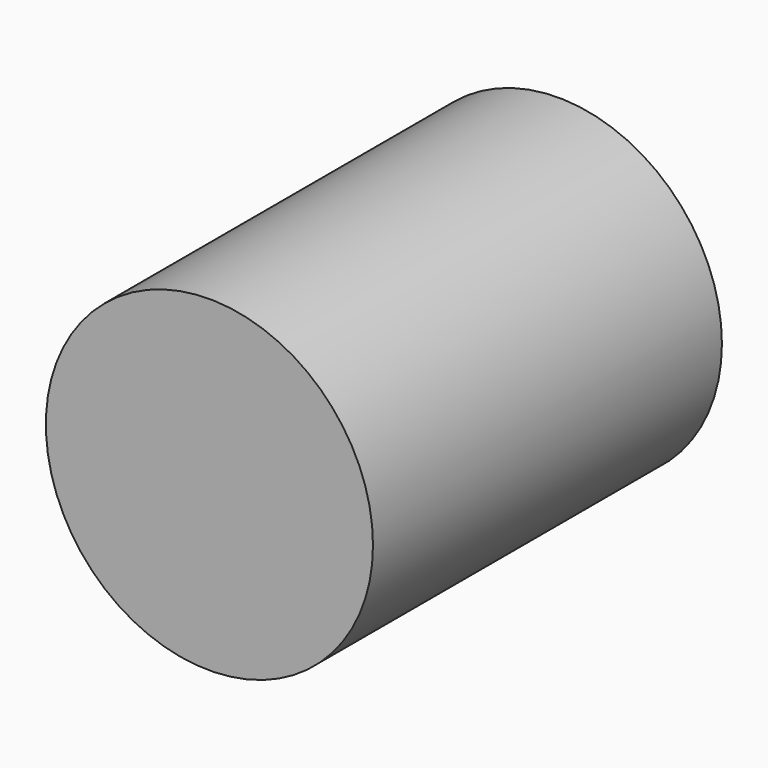
from build123d import *

# Parameters (mm, degrees)
F0_R     = 38.1
F0_R_2   = 19.05
F1_DEPTH = 50.8


# Not quite as in the source:
# - the program builds the solid bodies; features that only make, move or delete a surface that nothing else refers to are left out


with BuildPart() as f1:
    # F0 (on Front) → F1 (new body, symmetric)
    with BuildSketch(Plane.XZ):
        Circle(F0_R)
        Circle(F0_R_2, mode=Mode.SUBTRACT)
        Circle(F0_R_2)
    extrude(amount=F1_DEPTH, both=True)


solid = f1.part
